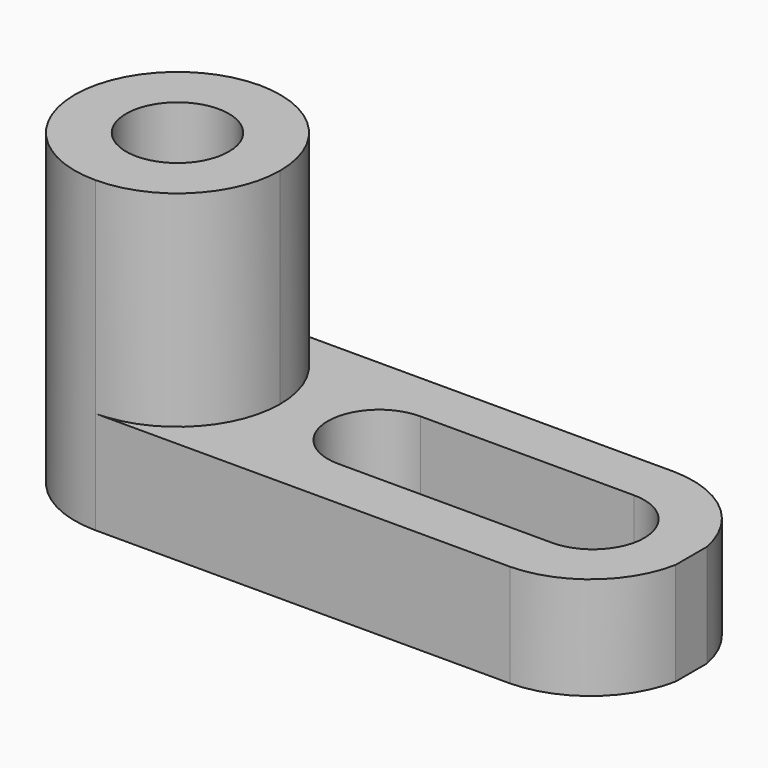
from build123d import *

# Parameters (mm, degrees)
F1_DEPTH = 25.4
F3_DEPTH = 12.701
F4_R     = 6.35
F5_DEPTH = 38.101
F7_DEPTH = 25.4


with BuildPart() as f1:
    # F0 (on Front) → F1 (new body)
    with BuildSketch(Plane.XZ):
        Polygon((-54.9375581781, 38.1), (-80.3375581781, 38.1), (-80.3375581781, 0), (-4.1375581781, 0), (-4.1375581781, 12.7), (-54.9375581781, 12.7), align=None)
    extrude(amount=F1_DEPTH)

    # F2 (on face) → F3 (cut, through all)
    with BuildSketch(Plane.XY.offset(12.7)):
        with BuildLine():
            ThreePointArc((-36.4283830897, -12.6069579273), (-38.2882550292, -8.1168298668), (-42.7783830897, -6.2569579273))
            ThreePointArc((-42.7783830897, -6.2569579273), (-49.1283830897, -12.6069579273), (-42.7783830897, -18.9569579273))
            ThreePointArc((-42.7783830897, -18.9569579273), (-38.2882550292, -17.0970859879), (-36.4283830897, -12.6069579273))
        make_face()
        with BuildLine():
            ThreePointArc((-16.3607828855, -18.9569579273), (-22.7107828855, -12.6069579273), (-16.3607828855, -6.2569579273))
            Line((-16.3607828855, -6.2569579273), (-42.7783830897, -6.2569579273))
            ThreePointArc((-42.7783830897, -6.2569579273), (-38.2882550292, -8.1168298668), (-36.4283830897, -12.6069579273))
            ThreePointArc((-36.4283830897, -12.6069579273), (-38.2882550292, -17.0970859879), (-42.7783830897, -18.9569579273))
            Line((-42.7783830897, -18.9569579273), (-16.3607828855, -18.9569579273))
        make_face()
        with BuildLine():
            ThreePointArc((-16.3607828855, -18.9569579273), (-11.870654825, -17.0970859879), (-10.0107828855, -12.6069579273))
            ThreePointArc((-10.0107828855, -12.6069579273), (-11.870654825, -8.1168298668), (-16.3607828855, -6.2569579273))
            ThreePointArc((-16.3607828855, -6.2569579273), (-22.7107828855, -12.6069579273), (-16.3607828855, -18.9569579273))
        make_face()
        with BuildLine():
            ThreePointArc((-16.3607828855, 0), (-8.4297023381, -2.981044621), (-4.1375581781, -10.2862594838))
            Line((-4.1375581781, -10.2862594838), (-4.1375581781, 0))
            Line((-4.1375581781, 0), (-16.3607828855, 0))
        make_face()
        with BuildLine():
            ThreePointArc((-4.1375581781, -15.1137405162), (-8.4297023381, -22.418955379), (-16.3607828855, -25.4))
            Line((-16.3607828855, -25.4), (-4.1375581781, -25.4))
            Line((-4.1375581781, -25.4), (-4.1375581781, -15.1137405162))
        make_face()
    extrude(amount=-F3_DEPTH, mode=Mode.SUBTRACT)

    # F4 (on face) → F5 (cut, through all)
    with BuildSketch(Plane.XY.offset(38.1)):
        with BuildLine():
            ThreePointArc((-80.3375581781, -12.7), (-76.6178142992, -3.7197438789), (-67.6375581781, 0))
            Line((-67.6375581781, 0), (-80.3375581781, 0))
            Line((-80.3375581781, 0), (-80.3375581781, -12.7))
        make_face()
        with BuildLine():
            Line((-80.3375581781, -25.4), (-67.6375581781, -25.4))
            ThreePointArc((-67.6375581781, -25.4), (-76.6178142992, -21.6802561211), (-80.3375581781, -12.7))
            Line((-80.3375581781, -12.7), (-80.3375581781, -25.4))
        make_face()
        with Locations((-67.6375581781, -12.7)):
            Circle(F4_R)
    extrude(amount=-F5_DEPTH, mode=Mode.SUBTRACT)

    # F6 (on face) → F7 (cut)
    with BuildSketch(Plane.XY.offset(38.1)):
        with BuildLine():
            ThreePointArc((-54.9375581781, -12.7), (-58.657302057, -21.6802561211), (-67.6375581781, -25.4))
            Line((-67.6375581781, -25.4), (-54.9375581781, -25.4))
            Line((-54.9375581781, -25.4), (-54.9375581781, -12.7))
        make_face()
        with BuildLine():
            ThreePointArc((-67.6375581781, 0), (-58.657302057, -3.7197438789), (-54.9375581781, -12.7))
            Line((-54.9375581781, -12.7), (-54.9375581781, 0))
            Line((-54.9375581781, 0), (-67.6375581781, 0))
        make_face()
    extrude(amount=-F7_DEPTH, mode=Mode.SUBTRACT)


solid = f1.part
